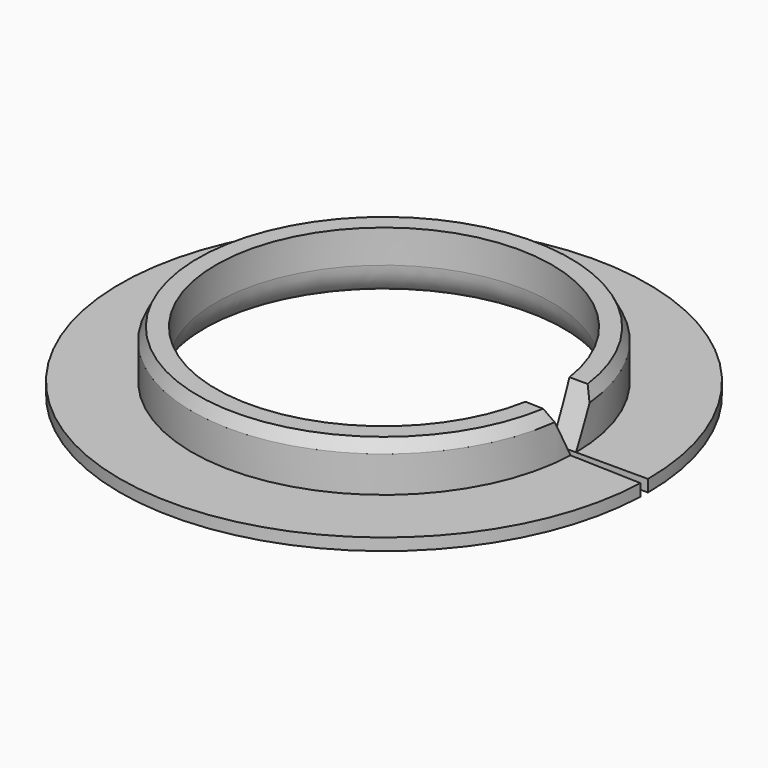
from build123d import *

# Parameters (mm, degrees)
F1_ANGLE    = 358
F2_C1_SIZE2 = 4
F2_C1_SIZE  = 2
F2_C2_SIZE2 = 4
F2_C2_SIZE  = 2
F3_SIZE     = 1
F4_R        = 3
F5_T2_ANGLE = 359.64


# Not quite as in the source:
# - a fillet or chamfer that OpenCascade refuses, or shapes differently, is made with other operations: its cross-section is extruded or revolved along the edge and cut away or added


with BuildPart() as f1:
    # F0 (on Front) → F1 (revolve)
    with BuildSketch(Plane.XZ):
        Polygon((14, 0), (22, 0), (22, 1), (16, 1), (16, 5), (14, 5), align=None)
    revolve(axis=Axis((0, 0, -0.0525576656), (0, 0, 1)), revolution_arc=F1_ANGLE)

    # F2: chamfer of 4 x 2 on 2 edges, made by hand

    # F2_c1
    f2_c1_edges = [f1.edges().sort_by_distance(p)[0] for p in [
        (15, 0, 5),
    ]]
    f2_c1_side = f1.faces().sort_by_distance((15, 0.04, 5))[0]
    chamfer(f2_c1_edges, length=F2_C1_SIZE, length2=F2_C1_SIZE2, reference=f2_c1_side)

    # F2_c2
    f2_c2_edges = [f1.edges().sort_by_distance(p)[0] for p in [
        (14.9908624053, -0.5234924505, 5),
    ]]
    f2_c2_side = f1.faces().sort_by_distance((14.9894664254, -0.5634680836, 5))[0]
    chamfer(f2_c2_edges, length=F2_C2_SIZE, length2=F2_C2_SIZE2, reference=f2_c2_side)

    # F3
    f3_edges = [f1.edges().sort_by_distance(p)[0] for p in [
        (-13.997868, 0.244334, 0),
    ]]
    chamfer(f3_edges, length=F3_SIZE)

    # F4
    f4_edges = [f1.edges().sort_by_distance(p)[0] for p in [
        (-13.997868, 0.244334, 1),
    ]]
    fillet(f4_edges, radius=F4_R)

    # F5: chamfer of 1 x 0.5 on 1 edges, made by hand

    # F5_s1 → F5_t2 (revolve, cut)
    with BuildSketch(Plane(origin=(0, 0, 0), x_dir=(0, 0, 1), z_dir=(-0.0143112113, -0.9998975894, 0))):
        Polygon((5, -15.5), (4, -16), (5, -16), align=None)
    revolve(axis=Axis((0, 0, 5), (0, 0, 1)), revolution_arc=F5_T2_ANGLE, mode=Mode.SUBTRACT)


solid = f1.part
